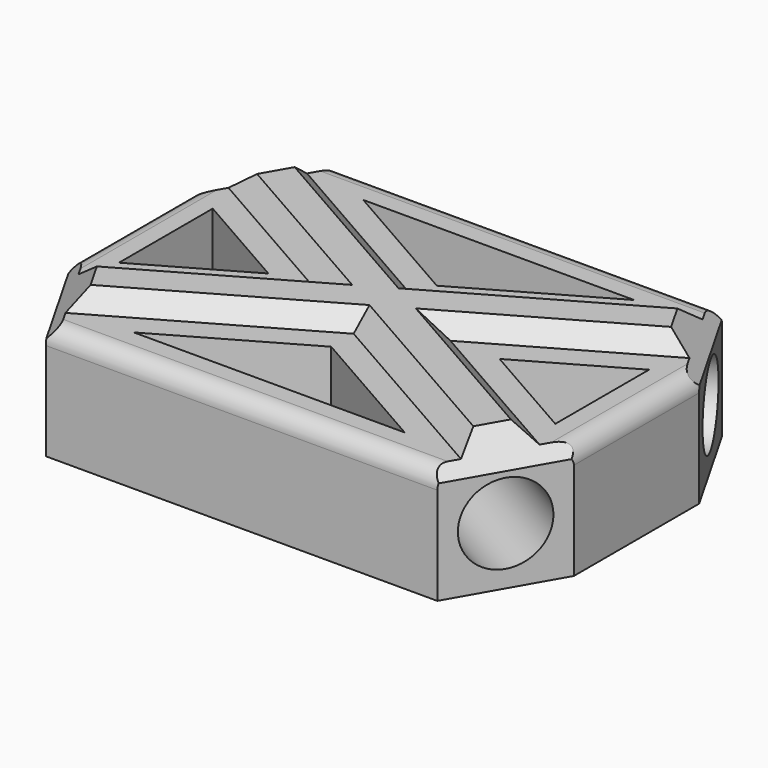
from build123d import *

# Parameters (mm, degrees)
F1_DEPTH      = 20
F2_R          = 7
F3_DEPTH      = 98.6163846154
F3_DEPTH_BACK = 8.6163846154
F4_R          = 7
F5_DEPTH      = 98.6163846154
F5_DEPTH_BACK = 8.6163846154
F7_DEPTH      = 3
F8_T4_DEPTH   = 57.4298435113
F8_T9_DEPTH   = 57.4298435113
F8_T14_DEPTH  = 56.5459149398
F8_T19_DEPTH  = 56.5459149398
F8_T24_DEPTH  = 56.5459149398
F8_T29_DEPTH  = 56.5459149398
F8_T34_DEPTH  = 57.4298435113
F8_T39_DEPTH  = 57.4298435113
F9_T1_DEPTH   = 31.2168298797
F9_T3_DEPTH   = 31.2168298797
F9_T5_DEPTH   = 31.2168298797
F10_R         = 3


# Not quite as in the source:
# - a fillet or chamfer that OpenCascade refuses, or shapes differently, is made with other operations: its cross-section is extruded or revolved along the edge and cut away or added


with BuildPart() as f1:
    # F0 (on Top) → F1 (new body)
    with BuildSketch(Plane.XY):
        Polygon((-23.609552012, 25.0086836473), (0, 25.0086836473), (23.609552012, 25.0086836473), (34.109552012, 31.0086836473), (-34.109552012, 31.0086836473), align=None)
        Polygon((0, 11.517511069), (-23.609552012, 25.0086836473), (-34.109552012, 31.0086836473), (-44.0323307792, 13.6438208048), (-38.0323307792, 10.2152493762), (-20.1556443707, 0), align=None)
        Polygon((34.109552012, 31.0086836473), (23.609552012, 25.0086836473), (0, 11.517511069), (20.1556443707, 0), (38.0323307792, 10.2152493762), (44.0323307792, 13.6438208048), align=None)
        Polygon((-38.0323307792, 10.2152493762), (-44.0323307792, 13.6438208048), (-44.0323307792, -13.6438208048), (-38.0323307792, -10.2152493762), (-38.0323307792, 0), align=None)
        Polygon((0, -11.517511069), (-20.1556443707, 0), (-38.0323307792, -10.2152493762), (-44.0323307792, -13.6438208048), (-34.109552012, -31.0086836473), (-23.609552012, -25.0086836473), align=None)
        Polygon((38.0323307792, -10.2152493762), (20.1556443707, 0), (0, -11.517511069), (23.609552012, -25.0086836473), (34.109552012, -31.0086836473), (44.0323307792, -13.6438208048), align=None)
        Polygon((44.0323307792, -13.6438208048), (44.0323307792, 13.6438208048), (38.0323307792, 10.2152493762), (38.0323307792, 0), (38.0323307792, -10.2152493762), align=None)
        Polygon((-23.609552012, -25.0086836473), (-34.109552012, -31.0086836473), (34.109552012, -31.0086836473), (23.609552012, -25.0086836473), (0, -25.0086836473), align=None)
        Polygon((20.1556443707, 0), (0, 11.517511069), (-20.1556443707, 0), (0, -11.517511069), align=None)
    extrude(amount=F1_DEPTH)

    # F2 (on face) → F3 (cut, two sides)
    with BuildSketch(Plane(origin=(-39.0709413956, -22.3262522261, 0), x_dir=(0.4961389384, -0.8682431421, 0), z_dir=(-0.8682431421, -0.4961389384, 0))) as f3_sk:
        with Locations((0, 10)):
            Circle(F2_R)
    extrude(amount=-F3_DEPTH, mode=Mode.SUBTRACT)
    extrude(f3_sk.sketch, amount=F3_DEPTH_BACK, mode=Mode.SUBTRACT)

    # F4 (on face) → F5 (cut, two sides)
    with BuildSketch(Plane(origin=(39.0709413956, -22.3262522261, 0), x_dir=(0.4961389384, 0.8682431421, 0), z_dir=(0.8682431421, -0.4961389384, 0))) as f5_sk:
        with Locations((0, 10)):
            Circle(F4_R)
    extrude(amount=-F5_DEPTH, mode=Mode.SUBTRACT)
    extrude(f5_sk.sketch, amount=F5_DEPTH_BACK, mode=Mode.SUBTRACT)

    # F6 (on face) → F7 (join)
    with BuildSketch(Plane.XY.offset(20)):
        Polygon((0, 0.8638133302), (-38.6988371918, 22.9774345827), (-39.0709413956, 22.3262522261), (-39.4430455994, 21.6750698695), (-1.5116733278, 0), align=None)
        Polygon((38.6988371918, 22.9774345827), (0, 0.8638133302), (1.5116733278, 0), (39.4430455994, 21.6750698695), (39.0709413956, 22.3262522261), align=None)
        Polygon((1.5116733278, 0), (0, 0.8638133302), (-1.5116733278, 0), (0, -0.8638133302), align=None)
        Polygon((39.4430455994, -21.6750698695), (1.5116733278, 0), (0, -0.8638133302), (38.6988371918, -22.9774345827), (39.0709413956, -22.3262522261), align=None)
        Polygon((0, -0.8638133302), (-1.5116733278, 0), (-39.4430455994, -21.6750698695), (-39.0709413956, -22.3262522261), (-38.6988371918, -22.9774345827), align=None)
    extrude(amount=F7_DEPTH)

    # F8: chamfer of 5 on 8 edges, made by hand


with BuildPart() as f8_tool2:
    # F8_s3 → F8_t4 (new body)
    with BuildSketch(Plane(origin=(-39.0709413956, -22.3262522261, 0), x_dir=(0, 0, 1), z_dir=(0.8682431421, 0.4961389384, 0))):
        Polygon((20, 5.75), (25, 0.75), (20, 0.75), align=None)
    extrude(amount=F8_T4_DEPTH)

    split(bisect_by=Plane.XY.offset(23), keep=Keep.BOTTOM)


with BuildPart() as f1_1:
    add(f1.part)

    # F8_t1: union F8_tool2
    add(f8_tool2.part)


with BuildPart() as f8_tool7:
    # F8_s8 → F8_t9 (new body)
    with BuildSketch(Plane(origin=(-10.7921263863, 6.1669293636, 0), x_dir=(0, 0, 1), z_dir=(0.8682431421, -0.4961389384, 0))):
        Polygon((20, 5.75), (25, 0.75), (20, 0.75), align=None)
    extrude(amount=F8_T9_DEPTH)

    split(bisect_by=Plane.XY.offset(23), keep=Keep.BOTTOM)


with BuildPart() as f1_2:
    add(f1_1.part)

    # F8_t6: union F8_tool7
    add(f8_tool7.part)


with BuildPart() as f8_tool12:
    # F8_s13 → F8_t14 (new body)
    with BuildSketch(Plane(origin=(10.0246614661, 5.7283779806, 0), x_dir=(0, 0, 1), z_dir=(-0.8682431421, -0.4961389384, 0))):
        Polygon((20, 5.75), (25, 0.75), (20, 0.75), align=None)
    extrude(amount=F8_T14_DEPTH)

    split(bisect_by=Plane.XY.offset(23), keep=Keep.BOTTOM)


with BuildPart() as f1_3:
    add(f1_2.part)

    # F8_t11: union F8_tool12
    add(f8_tool12.part)


with BuildPart() as f8_tool17:
    # F8_s18 → F8_t19 (new body)
    with BuildSketch(Plane(origin=(-39.0709413956, 22.3262522261, 0), x_dir=(0, 0, 1), z_dir=(0.8682431421, -0.4961389384, 0))):
        Polygon((20, 5.75), (25, 0.75), (20, 0.75), align=None)
    extrude(amount=F8_T19_DEPTH)

    split(bisect_by=Plane.XY.offset(23), keep=Keep.BOTTOM)


with BuildPart() as f1_4:
    add(f1_3.part)

    # F8_t16: union F8_tool17
    add(f8_tool17.part)


with BuildPart() as f8_tool22:
    # F8_s23 → F8_t24 (new body)
    with BuildSketch(Plane(origin=(39.0709413956, -22.3262522261, 0), x_dir=(0, 0, 1), z_dir=(-0.8682431421, 0.4961389384, 0))):
        Polygon((20, 5.75), (25, 0.75), (20, 0.75), align=None)
    extrude(amount=F8_T24_DEPTH)

    split(bisect_by=Plane.XY.offset(23), keep=Keep.BOTTOM)


with BuildPart() as f1_5:
    add(f1_4.part)

    # F8_t21: union F8_tool22
    add(f8_tool22.part)


with BuildPart() as f8_tool27:
    # F8_s28 → F8_t29 (new body)
    with BuildSketch(Plane(origin=(-10.0246614661, -5.7283779806, 0), x_dir=(0, 0, 1), z_dir=(0.8682431421, 0.4961389384, 0))):
        Polygon((20, 5.75), (25, 0.75), (20, 0.75), align=None)
    extrude(amount=F8_T29_DEPTH)

    split(bisect_by=Plane.XY.offset(23), keep=Keep.BOTTOM)


with BuildPart() as f1_6:
    add(f1_5.part)

    # F8_t26: union F8_tool27
    add(f8_tool27.part)


with BuildPart() as f8_tool32:
    # F8_s33 → F8_t34 (new body)
    with BuildSketch(Plane(origin=(10.7921263863, -6.1669293636, 0), x_dir=(0, 0, 1), z_dir=(-0.8682431421, 0.4961389384, 0))):
        Polygon((20, 5.75), (25, 0.75), (20, 0.75), align=None)
    extrude(amount=F8_T34_DEPTH)

    split(bisect_by=Plane.XY.offset(23), keep=Keep.BOTTOM)


with BuildPart() as f1_7:
    add(f1_6.part)

    # F8_t31: union F8_tool32
    add(f8_tool32.part)


with BuildPart() as f8_tool37:
    # F8_s38 → F8_t39 (new body)
    with BuildSketch(Plane(origin=(39.0709413956, 22.3262522261, 0), x_dir=(0, 0, 1), z_dir=(-0.8682431421, -0.4961389384, 0))):
        Polygon((20, 5.75), (25, 0.75), (20, 0.75), align=None)
    extrude(amount=F8_T39_DEPTH)

    split(bisect_by=Plane.XY.offset(23), keep=Keep.BOTTOM)


with BuildPart() as f1_8:
    add(f1_7.part)

    # F8_t36: union F8_tool37
    add(f8_tool37.part)

    # F9: chamfer of 5 on 4 edges, made by hand

    # F9_s2 → F9_t1 (cut)
    with BuildSketch(Plane(origin=(7.7439424177, -13.5518992309, 0), x_dir=(0, 0, 1), z_dir=(-0.4961389384, 0.8682431421, 0))):
        Polygon((18, -45), (23, -40), (23, -45), align=None)
        Polygon((18, 45), (23, 40), (23, 45), align=None)
    extrude(amount=F9_T1_DEPTH, mode=Mode.SUBTRACT)

    # F9_s4 → F9_t3 (cut)
    with BuildSketch(Plane(origin=(7.7439424177, 13.5518992309, 0), x_dir=(0, 0, 1), z_dir=(-0.4961389384, -0.8682431421, 0))):
        Polygon((18, 45), (23, 40), (23, 45), align=None)
    extrude(amount=F9_T3_DEPTH, mode=Mode.SUBTRACT)

    # F9_s6 → F9_t5 (cut)
    with BuildSketch(Plane(origin=(-7.7439424177, -13.5518992309, 0), x_dir=(0, 0, 1), z_dir=(0.4961389384, 0.8682431421, 0))):
        Polygon((18, 45), (23, 40), (23, 45), align=None)
    extrude(amount=F9_T5_DEPTH, mode=Mode.SUBTRACT)

    # F10
    f10_edges = [f1_8.edges().sort_by_distance(p)[0] for p in [
        (0, 31.008684, 20),
        (0, -31.008684, 20),
        (-44.032331, 0, 20),
        (44.032331, 0, 20),
    ]]
    fillet(f10_edges, radius=F10_R)


solid = f1_8.part
